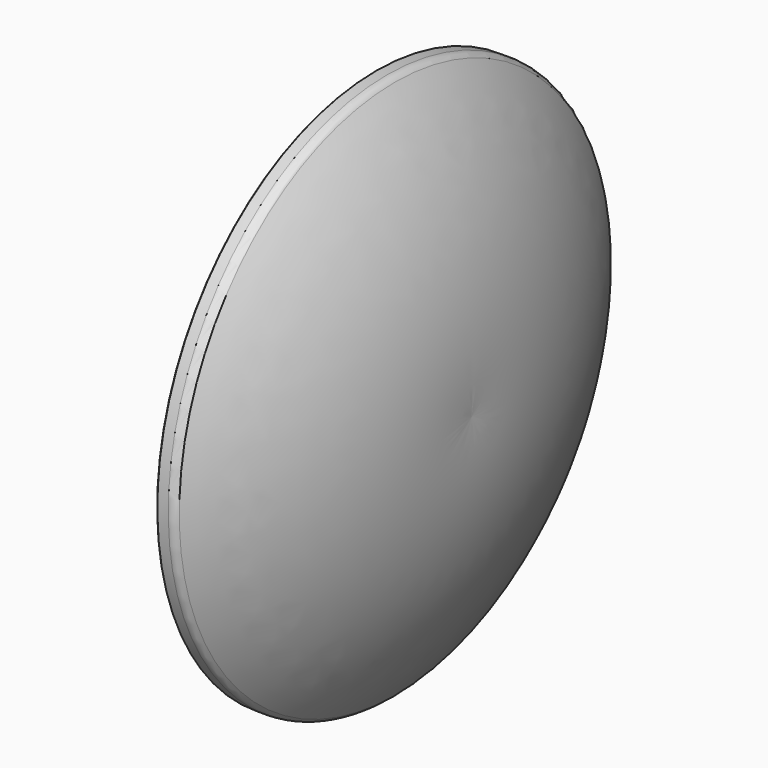
from build123d import *

# Parameters (mm, degrees)
F2_SIZE = 5


with BuildPart() as f1:
    # F0 (on Front) → F1 (revolve)
    with BuildSketch(Plane.XZ):
        with BuildLine():
            Line((979.6323661451, 2000), (895, 2000))
            Line((895, 2000), (895, 1985))
            Line((895, 1985), (979.6323661451, 1985))
            ThreePointArc((979.6323661451, 1985), (1004.6928400922, 1978.9588872989), (1024.2481086772, 1962.1626416562))
            ThreePointArc((1024.2481086772, 1962.1626416562), (1474.8680375413, 1030.0104667169), (1579.9605491074, 0))
            Line((1579.9605491074, 0), (1595, 0))
            ThreePointArc((1595, 0), (1489.1516471948, 1034.6229244194), (1036.4160384587, 1970.9342711989))
            ThreePointArc((1036.4160384587, 1970.9342711989), (1011.5275148051, 1992.3113111077), (979.6323661451, 2000))
        make_face()
    revolve(axis=Axis((1245, 0, 0), (-1, 0, 0)))

    # F2
    f2_edges = [f1.edges().sort_by_distance(p)[0] for p in [
        (895, 0, -2000),
        (895, 0, -1985),
    ]]
    chamfer(f2_edges, length=F2_SIZE)


solid = f1.part
